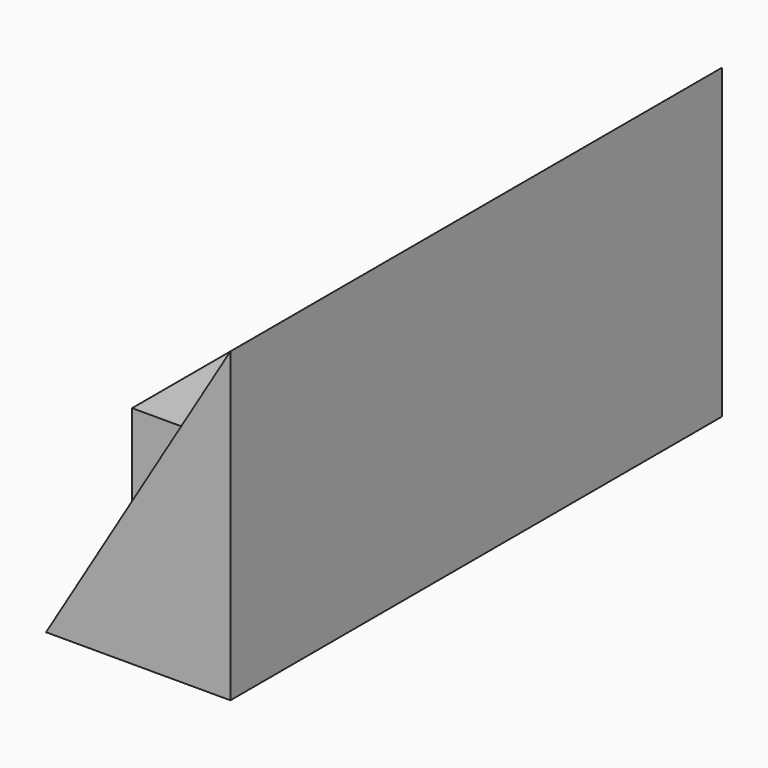
from build123d import *

# Parameters (mm, degrees)
F1_DEPTH = 127
F2_START = 22.225
F2_DEPTH = 82.55


# Not quite as in the source:
# - a length typed as a fraction of an inch, garbled in the dataset ("3 / 203.2 mm" for 3/8 in), is restored


with BuildPart() as f1:
    # F0 (on Front) → F1 (new body)
    with BuildSketch(Plane.XZ):
        Polygon((-22.9990067312, -31.75), (-22.9990067312, 31.75), (-42.0490067312, 0), (-61.0990067312, -31.75), align=None)
    extrude(amount=F1_DEPTH)

    # F0 (on Front) → F2 (join)
    with BuildSketch(Plane.XZ.offset(F2_START)):
        Polygon((-61.0990067312, -31.75), (-42.0490067312, 0), (-61.0990067312, 0), align=None)
    extrude(amount=F2_DEPTH)


solid = f1.part
